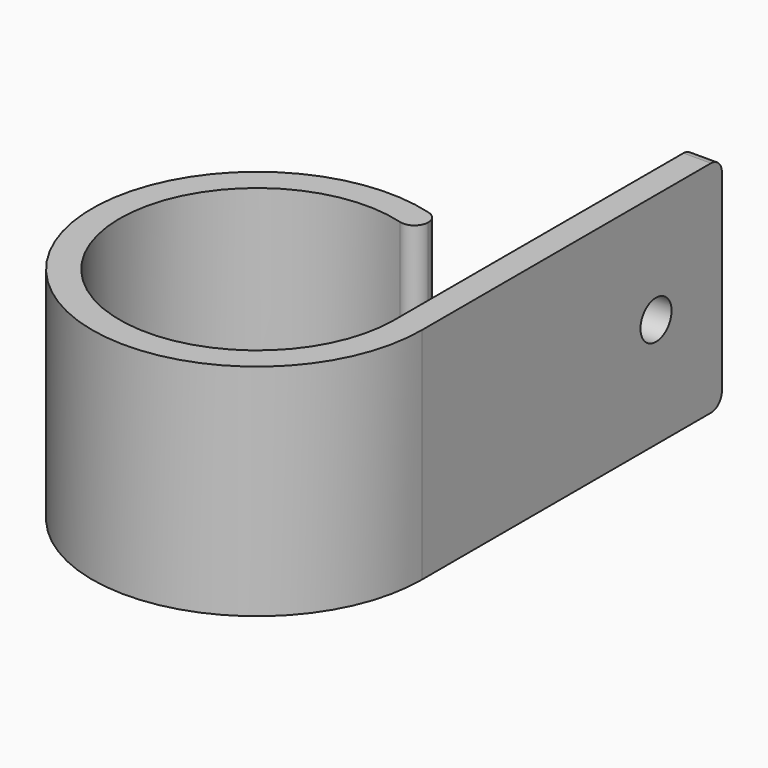
from build123d import *

# Parameters (mm, degrees)
F1_DEPTH = 12.7
F2_R     = 1.58749
F3_R     = 1.5875
F5_D     = 4.4958


# Not quite as in the source:
# - a fillet or chamfer is up to 0.001 mm smaller than in the source, because OpenCascade refuses the exact size


with BuildPart() as f1:
    # F0 (on Top) → F1 (new body, symmetric)
    with BuildSketch(Plane.XY):
        with BuildLine():
            Line((0, 43.3605122421), (0, 0))
            ThreePointArc((0, 0), (-29.1569779212, -8.6950956004), (-9.525, 14.5496778315))
            Line((-9.525, 14.5496778315), (-9.525, 17.9605122421))
            ThreePointArc((-9.525, 17.9605122421), (-31.4292598667, -10.9985226281), (3.175, 0))
            Line((3.175, 0), (3.175, 43.3605122421))
            Line((3.175, 43.3605122421), (0, 43.3605122421))
        make_face()
    extrude(amount=F1_DEPTH, both=True)

    # F2 (radius 1.5875 in the source; OpenCascade refuses exactly that, so slightly less here)
    f2_edges = [f1.edges().sort_by_distance(p)[0] for p in [
        (-9.525, 14.549678, 0),
        (-9.525, 17.960512, 0),
    ]]
    fillet(f2_edges, radius=F2_R)

    # F3
    f3_edges = [f1.edges().sort_by_distance(p)[0] for p in [
        (1.5875, 43.360512, 12.7),
        (1.5875, 43.360512, -12.7),
    ]]
    fillet(f3_edges, radius=F3_R)

    # F5 (through all)
    with Locations(Plane(origin=(0, 0, 0), x_dir=(0, 1, 0), z_dir=(-1, 0, 0))):
        with Locations((33.8355122421, 0)):
            Hole(F5_D / 2)


solid = f1.part
